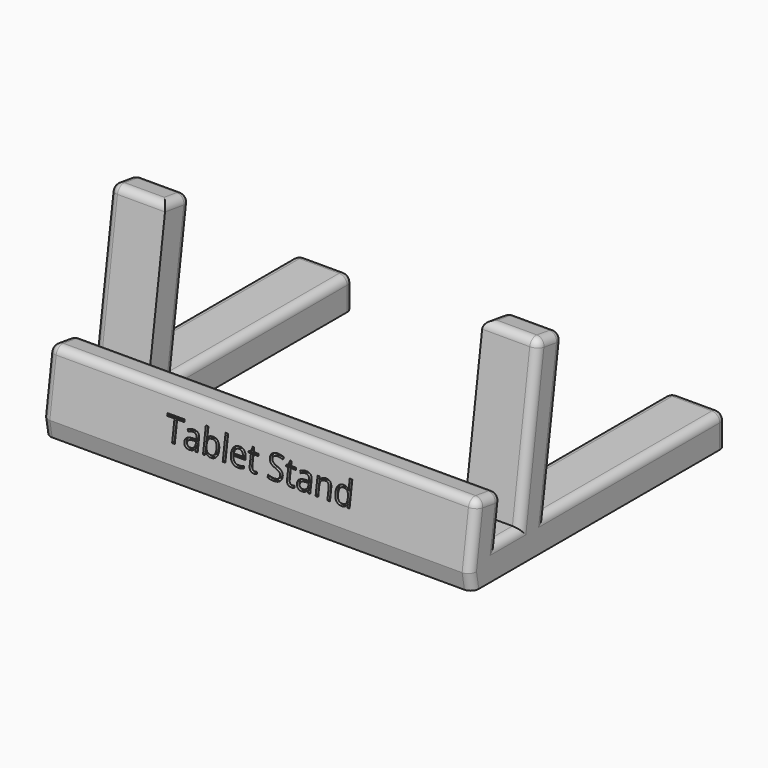
from build123d import *

# Parameters (mm, degrees)
F1_DEPTH     = 135
F3_DEPTH     = 109.2
F5_W         = 100
F5_H         = 34.8088418269
F6_DEPTH     = 25
F4_TEXT_SIZE = 10.1474669969
F7_DEPTH     = 1
F8_W         = 100
F8_H         = 42.1801268728
F9_DEPTH     = 25
F10_R        = 2.5


# Not quite as in the source:
# - Text() gives the source's letters only with a copy of the font that has no kerning and outlines rounded to 1/6400 em; it was checked with that copy


with BuildPart() as f1:
    # F0 (on Right) → F1 (new body)
    with BuildSketch(Plane.YZ):
        Polygon((-0.8972655273, 5.1302352849), (0, 0), (100, 0), (100, 10), (29.0191436607, 10), (35.9927355312, 58.045071606), (26.0964378799, 59.481488257), (18.9143546252, 10), (9.9143546252, 10), (11.8392316318, 23.2615810237), (1.9429339804, 24.6979976746), align=None)
    extrude(amount=F1_DEPTH)

    # F2 (on face) → F3 (cut)
    with BuildSketch(Plane(origin=(0, 17.102575436, -2.4823853319), x_dir=(1, 0, 0), z_dir=(0, -0.9896297651, 0.1436416651))):
        Polygon((117.5, 62.6131870439), (67.5, 62.6131870439), (17.5, 62.6131870439), (17.5, 12.6131870439), (117.5, 12.6131870439), align=None)
    extrude(amount=-F3_DEPTH, mode=Mode.SUBTRACT)

    # F5 (on face) → F6 (cut)
    with BuildSketch(Plane(origin=(0, 1.8117791891, 12.4823853319), x_dir=(1, 0, 0), z_dir=(0, 0.1436416651, 0.9896297651))):
        with Locations((67.5, 69.4950544149)):
            Rectangle(F5_W, F5_H)
    extrude(amount=-F6_DEPTH, mode=Mode.SUBTRACT)

    # F4 (on face) → F7 (cut)
    with BuildSketch(Plane(origin=(0, -1.6080258638, 0.2333999246), x_dir=(1, 0, 0), z_dir=(0, -0.9896297651, 0.1436416651))):
        with Locations((38.0089240403, 10.6648690999)):
            Text('Tablet Stand', F4_TEXT_SIZE, font='Open Sans', text_align=(TextAlign.LEFT, TextAlign.BOTTOM))
    extrude(amount=-F7_DEPTH, mode=Mode.SUBTRACT)

    # F8 (on face) → F9 (cut)
    with BuildSketch(Plane.XY.offset(10)):
        with Locations((67.5, 40.0044180616)):
            Rectangle(F8_W, F8_H)
    extrude(amount=-F9_DEPTH, mode=Mode.SUBTRACT)

    # F10
    f10_edges = [f1.edges().sort_by_distance(p)[0] for p in [
        (67.5, 1.942934, 24.697998),
        (67.5, 11.839232, 23.261581),
        (135, 22.505396, 34.740744),
        (135, 32.50594, 34.022536),
        (135, 14.414355, 10),
        (135, 10.876793, 16.630791),
        (135, 0.522834, 14.914116),
        (0, 0.522834, 14.914116),
        (0, -0.448633, 2.565118),
        (135, -0.448633, 2.565118),
        (0, 14.414355, 10),
        (0, 10.876793, 16.630791),
        (117.5, 32.50594, 34.022536),
        (135, 64.509572, 10),
        (117.5, 64.509572, 10),
        (17.5, 64.509572, 10),
        (0, 64.509572, 10),
        (17.5, 32.50594, 34.022536),
        (0, 32.50594, 34.022536),
        (0, 31.044587, 58.76328),
        (8.75, 26.096438, 59.481488),
        (17.5, 31.044587, 58.76328),
        (8.75, 35.992736, 58.045072),
        (126.25, 35.992736, 58.045072),
        (135, 31.044587, 58.76328),
        (126.25, 26.096438, 59.481488),
        (117.5, 31.044587, 58.76328),
        (0, 22.505396, 34.740744),
        (8.75, 100, 10),
        (17.5, 100, 5),
        (0, 100, 5),
        (117.5, 100, 5),
        (126.25, 100, 10),
        (135, 100, 5),
        (67.5, 18.914355, 10),
        (0, 6.891083, 23.979789),
        (135, 6.891083, 23.979789),
    ]]
    fillet(f10_edges, radius=F10_R)


solid = f1.part
